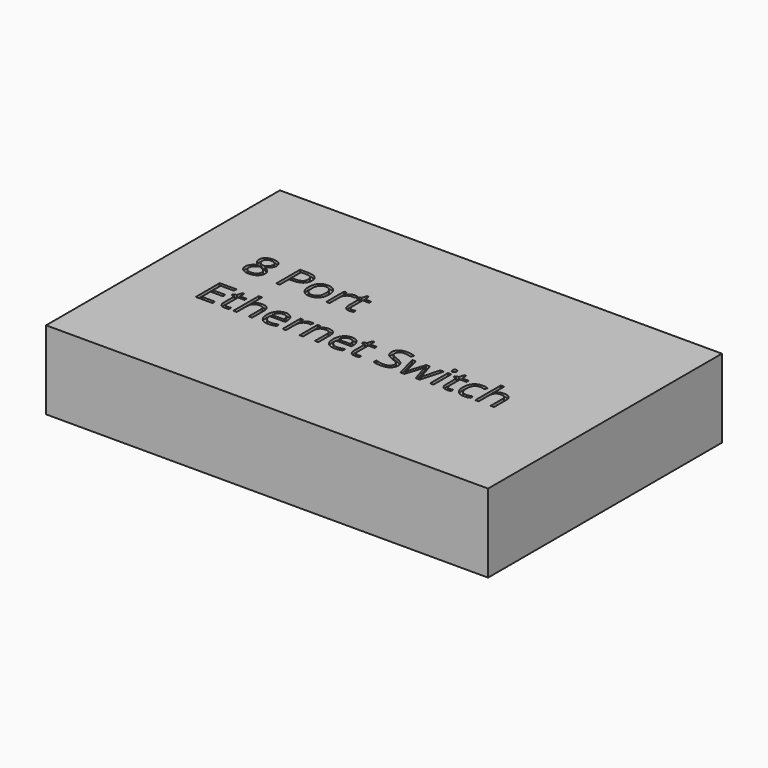
from build123d import *

# Parameters (mm, degrees)
F0_W         = 157.48
F0_H         = 104.14
F1_DEPTH     = 27.94
F2_TEXT_SIZE = 14.9147730554
F3_DEPTH     = 1


# Not quite as in the source:
# - Text() gives the source's letters only with a copy of the font that has no kerning and outlines rounded to 1/6400 em; it was checked with that copy


with BuildPart() as f1:
    # F0 (on Top) → F1 (new body)
    with BuildSketch(Plane.XY):
        Rectangle(F0_W, F0_H)
    extrude(amount=F1_DEPTH)

    # F2 (on face) → F3 (cut)
    with BuildSketch(Plane.XY.offset(27.94)):
        with Locations((-58.3700679445, 7.5993764913)):
            Text('8 Port', F2_TEXT_SIZE, font='Open Sans', text_align=(TextAlign.LEFT, TextAlign.BOTTOM))
        with Locations((-58.3700679445, -12.684714864)):
            Text('Ethernet Switch', F2_TEXT_SIZE, font='Open Sans', text_align=(TextAlign.LEFT, TextAlign.BOTTOM))
    extrude(amount=-F3_DEPTH, mode=Mode.SUBTRACT)


solid = f1.part
